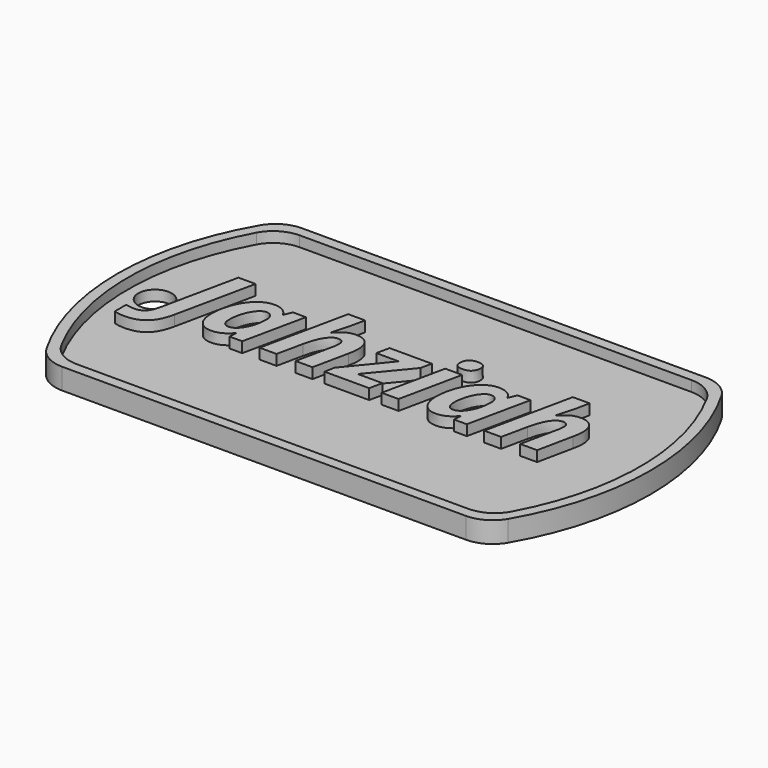
from build123d import *

# Parameters (mm, degrees)
F1_DEPTH     = 1
F3_DEPTH     = 1
F4_R         = 1.5875
F5_DEPTH     = 1
F6_TEXT_SIZE = 10.9737477032
F7_DEPTH     = 1


# Not quite as in the source:
# - Text() gives the source's letters only with a copy of the font that has no kerning and outlines rounded to 1/6400 em; it was checked with that copy


with BuildPart() as f1:
    # F0 (on Top) → F1 (new body)
    with BuildSketch(Plane.XY):
        with BuildLine():
            ThreePointArc((-19.2474145991, 14.2875), (-20.8349145991, 13.862130657), (-21.9970452561, 12.7))
            ThreePointArc((-21.9970452561, 12.7), (-25.4, 0), (-21.9970452561, -12.7))
            ThreePointArc((-21.9970452561, -12.7), (-20.8349145991, -13.862130657), (-19.2474145991, -14.2875))
            Line((-19.2474145991, -14.2875), (19.2474145991, -14.2875))
            ThreePointArc((19.2474145991, -14.2875), (20.8349145991, -13.862130657), (21.9970452561, -12.7))
            ThreePointArc((21.9970452561, -12.7), (25.4, 0), (21.9970452561, 12.7))
            ThreePointArc((21.9970452561, 12.7), (20.8349145991, 13.862130657), (19.2474145991, 14.2875))
            Line((19.2474145991, 14.2875), (-19.2474145991, 14.2875))
        make_face()
    extrude(amount=F1_DEPTH)

    # F2 (on face) → F3 (join)
    with BuildSketch(Plane.XY.offset(1)):
        with BuildLine():
            Line((19.2474145991, 14.2875), (-19.2474145991, 14.2875))
            ThreePointArc((-19.2474145991, 14.2875), (-20.8349145991, 13.862130657), (-21.9970452561, 12.7))
            ThreePointArc((-21.9970452561, 12.7), (-25.4, 0), (-21.9970452561, -12.7))
            ThreePointArc((-21.9970452561, -12.7), (-20.8349145991, -13.862130657), (-19.2474145991, -14.2875))
            Line((-19.2474145991, -14.2875), (19.2474145991, -14.2875))
            ThreePointArc((19.2474145991, -14.2875), (20.8349145991, -13.862130657), (21.9970452561, -12.7))
            ThreePointArc((21.9970452561, -12.7), (25.4, 0), (21.9970452561, 12.7))
            ThreePointArc((21.9970452561, 12.7), (20.8349145991, 13.862130657), (19.2474145991, 14.2875))
        make_face()
        with BuildLine():
            ThreePointArc((-21.4526124879, 11.6252061249), (-20.2856017842, 12.8404540819), (-18.6611352482, 13.2875))
            Line((-18.6611352482, 13.2875), (18.6611352482, 13.2875))
            ThreePointArc((18.6611352482, 13.2875), (20.2856017842, 12.8404540819), (21.4526124879, 11.6252061249))
            ThreePointArc((21.4526124879, 11.6252061249), (24.4, 0), (21.4526124879, -11.6252061249))
            ThreePointArc((21.4526124879, -11.6252061249), (20.2856017842, -12.8404540819), (18.6611352482, -13.2875))
            Line((18.6611352482, -13.2875), (-18.6611352482, -13.2875))
            ThreePointArc((-18.6611352482, -13.2875), (-20.2856017842, -12.8404540819), (-21.4526124879, -11.6252061249))
            ThreePointArc((-21.4526124879, -11.6252061249), (-24.4, 0), (-21.4526124879, 11.6252061249))
        make_face(mode=Mode.SUBTRACT)
    extrude(amount=F3_DEPTH)

    # F4 (on face) → F5 (cut)
    with BuildSketch(Plane.XY.offset(1)):
        with Locations((-21.821282804, 0)):
            Circle(F4_R)
    extrude(amount=-F5_DEPTH, mode=Mode.SUBTRACT)

    # F6 (on face) → F7 (join)
    with BuildSketch(Plane.XY.offset(1)):
        with Locations((-20.0322335027, -2.7130285744)):
            Text('Jahziah', F6_TEXT_SIZE, font='Open Sans', font_style=FontStyle.BOLDITALIC, text_align=(TextAlign.LEFT, TextAlign.BOTTOM))
    extrude(amount=F7_DEPTH)


solid = f1.part
